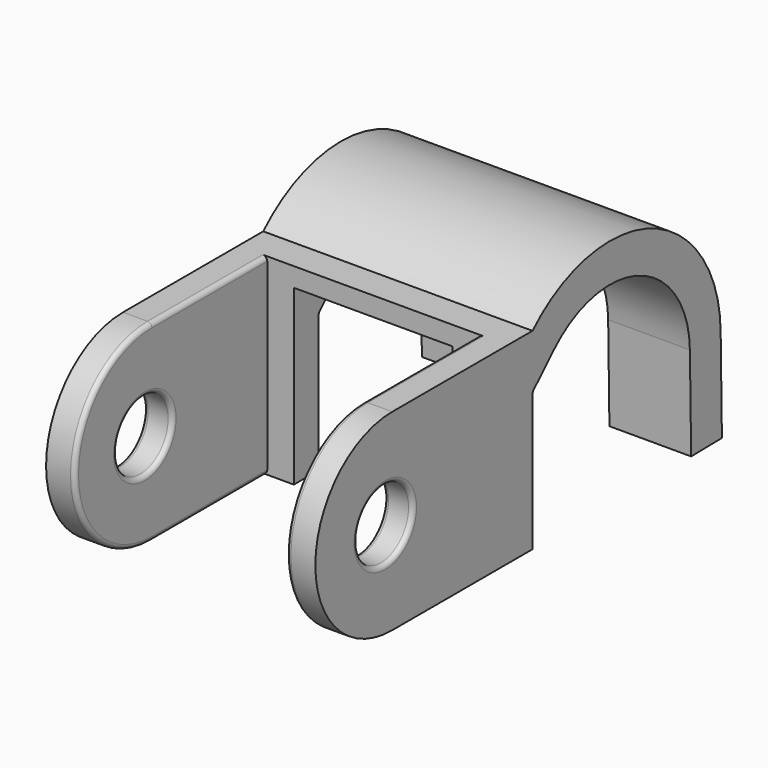
from build123d import *

# Parameters (mm, degrees)
F0_R     = 1.8
F1_DEPTH = 14
F2_W     = 5.5
F2_H     = 4.0708386075
F2_H_2   = 4.9094793208
F3_DEPTH = 5
F4_W     = 11
F4_H     = 7.5
F5_DEPTH = 12
F6_R     = 0.2312376478
F7_W     = 8.2372972146
F7_H     = 9.0102642961
F8_DEPTH = 5


# Not quite as in the source:
# - a feature names something its author has since deleted; it is built from what else it names


with BuildPart() as f1:
    # F0 (on Right) → F1 (new body)
    with BuildSketch(Plane.YZ):
        with BuildLine():
            Line((-9.1132364464, -5), (0, -5))
            Line((0, -5), (0, 2.1922827341))
            Line((0, 2.1922827341), (1.4037047395, 3.5753551798))
            ThreePointArc((1.4037047395, 3.5753551798), (7.0067613017, 4.6816844814), (10.2298574217, -0.0331706346))
            Line((10.2298574217, -0.0331706346), (10.3112826954, -4.9419746769))
            Line((10.3112826954, -4.9419746769), (12.3110075686, -4.9088040424))
            Line((12.3110075686, -4.9088040424), (12.2295822948, 0))
            ThreePointArc((12.2295822948, 0), (7.7636365241, 6.5329380451), (0, 5))
            Line((0, 5), (-9.1132364464, 5))
            ThreePointArc((-9.1132364464, 5), (-14.1132364464, 0), (-9.1132364464, -5))
        make_face()
        with Locations((-9.5687768728, 0)):
            Circle(F0_R, mode=Mode.SUBTRACT)
    extrude(amount=F1_DEPTH)

    # F2 (on face) → F3 (cut)
    with BuildSketch(Plane(origin=(0, 12.2262182699, 0.2028036077), x_dir=(-1, 0, 0), z_dir=(0, 0.9998624542, 0.0165853176))):
        with Locations((-7, 1.8325877974)):
            Rectangle(F2_W, F2_H)
        with Locations((-7, -2.6575711668)):
            Rectangle(F2_W, F2_H_2)
    extrude(amount=-F3_DEPTH, mode=Mode.SUBTRACT)

    # F4 (on face) → F5 (cut)
    with BuildSketch(Plane(origin=(0, 0, -5), x_dir=(1, 0, 0), z_dir=(0, 0, -1))):
        with Locations((7, 5.3632364464)):
            Rectangle(F4_W, F4_H)
        with Locations((7, 12.8632364464)):
            Rectangle(F4_W, F4_H)
    extrude(amount=-F5_DEPTH, mode=Mode.SUBTRACT)

    # F6
    f6_edges = [f1.edges().sort_by_distance(p)[0] for p in [
        (1.5, -11.368777, 0),
        (12.5, -11.368777, 0),
        (0, -11.368777, 0),
        (14, -11.368777, 0),
        (7, 0, 2.192283),
        (12.5, -5.363236, -5),
        (1.5, -5.363236, -5),
        (12.5, -14.113236, 0),
        (12.5, -5.363236, 5),
        (1.5, -5.363236, 5),
        (1.5, -14.113236, 0),
    ]]
    fillet(f6_edges, radius=F6_R)

    # F7 (on face) → F8 (cut)
    with BuildSketch(Plane.XZ.offset(1.6132364464)):
        with Locations((7, -0.494867852)):
            Rectangle(F7_W, F7_H)
    extrude(amount=-F8_DEPTH, mode=Mode.SUBTRACT)


with BuildPart() as f9_1:
    # F9: copy of F1
    add(f1.part)


with BuildPart() as f11_1:
    # F11: copy of F1
    add(f1.part)


solid = f1.part
